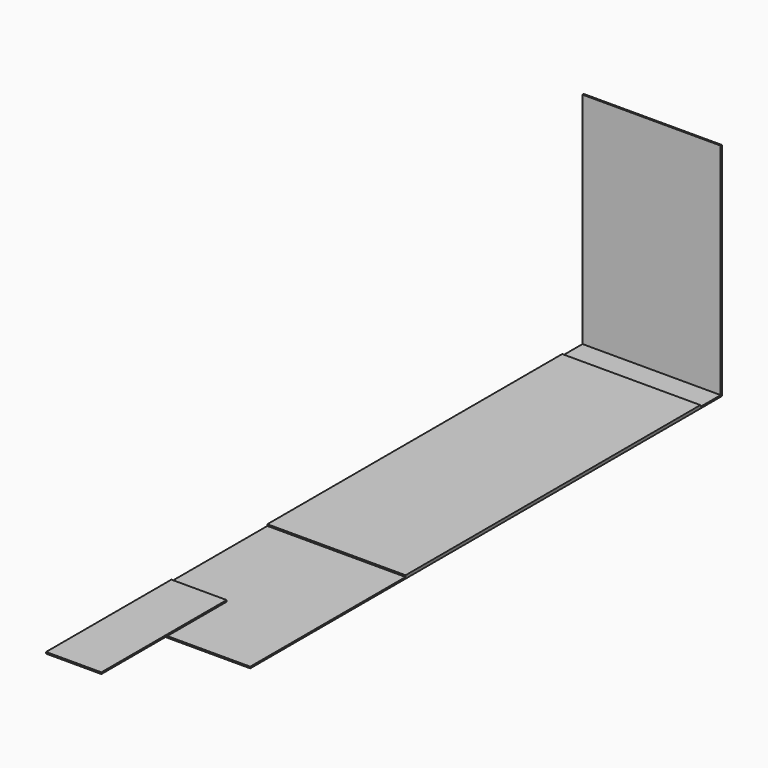
from build123d import *

# Parameters (mm, degrees)
F0_W     = 571.5
F0_H     = 2438.4
F1_DEPTH = 6.35
F2_W     = 571.5
F2_H     = 6.35
F3_DEPTH = 914.4
F4_W     = 228.6
F4_H     = 647.7
F5_DEPTH = 6.35
F6_W     = 571.5
F6_H     = 1524
F7_DEPTH = 6.35


# Not quite as in the source:
# - a length typed as a fraction of an inch, garbled in the dataset ("3 / 203.2 mm" for 3/8 in), is restored


with BuildPart() as f1:
    # F0 (on Top) → F1 (new body)
    with BuildSketch(Plane.XY):
        with Locations((285.75, -1219.2)):
            Rectangle(F0_W, F0_H)
    extrude(amount=F1_DEPTH)


with BuildPart() as f3:
    # F2 (on Top) → F3 (new body)
    with BuildSketch(Plane.XY):
        with Locations((285.75, -3.175)):
            Rectangle(F2_W, F2_H)
    extrude(amount=F3_DEPTH)


with BuildPart() as f5:
    # F4 (on face) → F5 (new body)
    with BuildSketch(Plane.XY.offset(6.35)):
        with Locations((114.3, -2455.4346443176)):
            Rectangle(F4_W, F4_H)
    extrude(amount=F5_DEPTH)


with BuildPart() as f7:
    # F6 (on face) → F7 (new body)
    with BuildSketch(Plane.XY.offset(6.35)):
        with Locations((285.75, -873.3578567505)):
            Rectangle(F6_W, F6_H)
    extrude(amount=F7_DEPTH)


solid = Compound([f1.part, f3.part, f5.part, f7.part])
